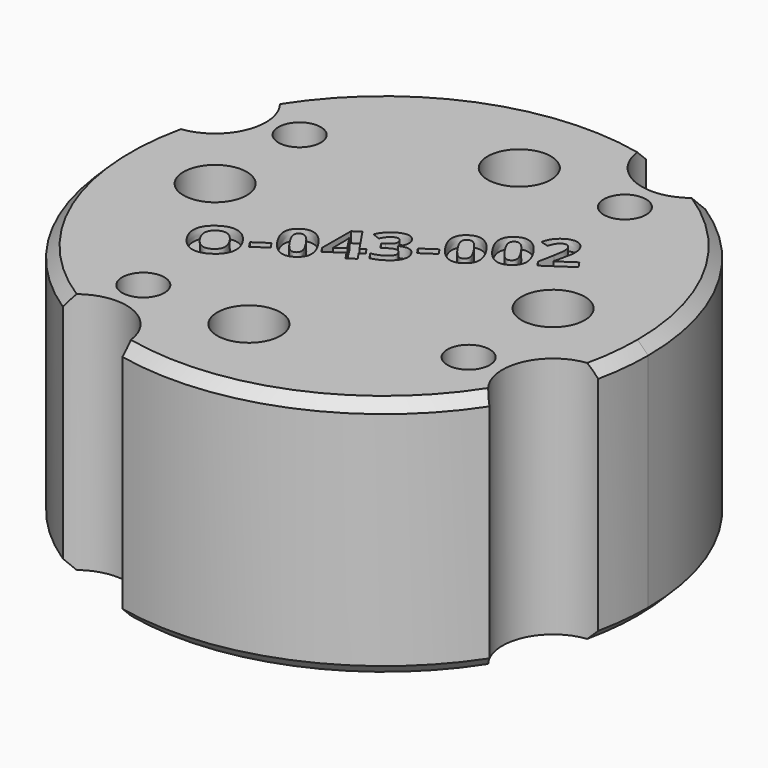
from build123d import *

# Parameters (mm, degrees)
F0_R         = 2
F0_R_2       = 3
F1_DEPTH     = 23
F2_TEXT_SIZE = 6.1259651586
F3_DEPTH     = 1
F4_SIZE      = 1


# Not quite as in the source:
# - a feature names something its author has since deleted; it is built from what else it names
# - Text() gives the source's letters only with a copy of the font that has no kerning and outlines rounded to 1/6400 em; it was checked with that copy


with BuildPart() as f1:
    # F0 (on Top) → F1 (new body)
    with BuildSketch(Plane.XY):
        with BuildLine():
            ThreePointArc((24.4487408728, -5.2210219054), (24.8618032514, -2.6250217314), (25, 0))
            ThreePointArc((25, 0), (21.9896884421, 11.8934268493), (13.6837118225, 20.922620074))
            ThreePointArc((13.6837118225, 20.922620074), (8.1538461538, 19.5692307692), (5.2210219054, 24.4487408728))
            ThreePointArc((5.2210219054, 24.4487408728), (-9.5187451314, 23.1169524619), (-20.922620074, 13.6837118225))
            ThreePointArc((-20.922620074, 13.6837118225), (-19.5692307692, 8.1538461538), (-24.4487408728, 5.2210219054))
            ThreePointArc((-24.4487408728, 5.2210219054), (-23.1169524619, -9.5187451314), (-13.6837118225, -20.922620074))
            ThreePointArc((-13.6837118225, -20.922620074), (-8.1538461538, -19.5692307692), (-5.2210219054, -24.4487408728))
            ThreePointArc((-5.2210219054, -24.4487408728), (9.5187451314, -23.1169524619), (20.922620074, -13.6837118225))
            ThreePointArc((20.922620074, -13.6837118225), (19.5692307692, -8.1538461538), (24.4487408728, -5.2210219054))
        make_face()
        with Locations((-10, -16)):
            Circle(F0_R, mode=Mode.SUBTRACT)
        with Locations((0, -16)):
            Circle(F0_R_2, mode=Mode.SUBTRACT)
        with Locations((16, -10)):
            Circle(F0_R, mode=Mode.SUBTRACT)
        with Locations((-16, 0)):
            Circle(F0_R_2, mode=Mode.SUBTRACT)
        with Locations((-16, 10)):
            Circle(F0_R, mode=Mode.SUBTRACT)
        with Locations((16, 0)):
            Circle(F0_R_2, mode=Mode.SUBTRACT)
        with Locations((0, 16)):
            Circle(F0_R_2, mode=Mode.SUBTRACT)
        with Locations((10, 16)):
            Circle(F0_R, mode=Mode.SUBTRACT)
    extrude(amount=F1_DEPTH)

    # F2 (on face) → F3 (cut)
    with BuildSketch(Plane.XY.offset(23)):
        with Locations(Location((-11.2023489406, -10.2162094545), (0, 0, 34))):
            Text('O-043-002', F2_TEXT_SIZE, font='Open Sans', font_style=FontStyle.BOLD, text_align=(TextAlign.LEFT, TextAlign.BOTTOM))
    extrude(amount=-F3_DEPTH, mode=Mode.SUBTRACT)

    # F4
    f4_edges = [f1.edges().sort_by_distance(p)[0] for p in [
        (-23.116952, -9.518745, 0),
        (-23.116952, -9.518745, 23),
        (9.518745, -23.116952, 0),
        (9.518745, -23.116952, 23),
        (23.116952, 9.518745, 23),
        (23.116952, 9.518745, 0),
        (-9.518745, 23.116952, 0),
        (-9.518745, 23.116952, 23),
    ]]
    chamfer(f4_edges, length=F4_SIZE)


solid = f1.part
